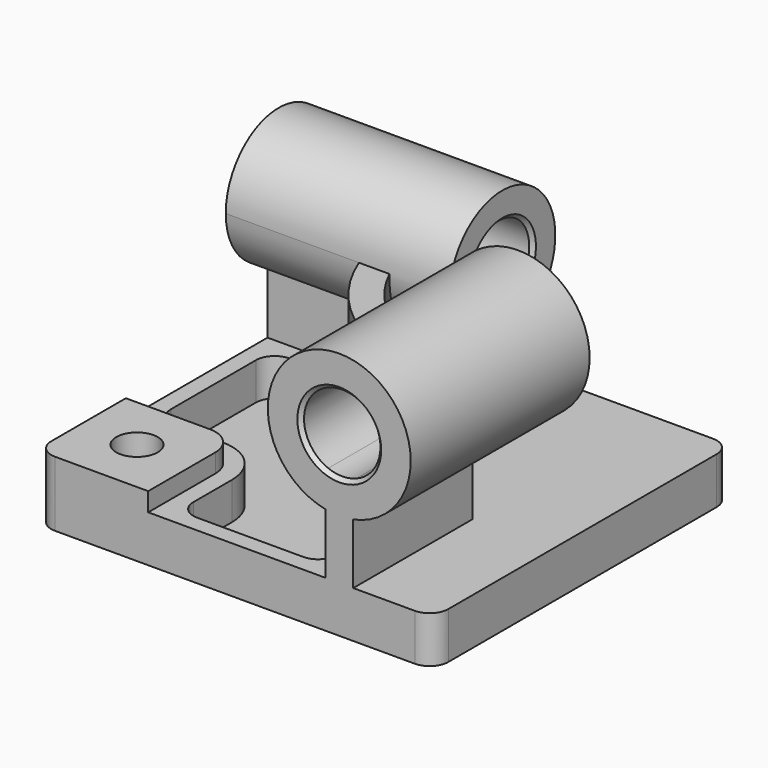
from build123d import *

# Parameters (mm, degrees)
F0_W            = 213
F0_H            = 25
F1_DEPTH        = 100
F3_DEPTH        = 20
F4_DEPTH        = 70
F5_R            = 38.333333335
F5_R_2          = 20.5
F6_DEPTH        = 120
F7_R            = 35.5
F7_R_2          = 20.5
F8_DEPTH        = 120
F9_DEPTH        = 213.001
F10_DEPTH       = 200.001
F11_DEPTH       = 10
F13_D           = 14.75
F13_CBORE_D     = 22.25
F13_CBORE_DEPTH = 14
F14_R           = 10


# Not quite as in the source:
# - a fillet or chamfer that OpenCascade refuses, or shapes differently, is made with other operations: its cross-section is extruded or revolved along the edge and cut away or added


with BuildPart() as f1:
    # F0 (on Front) → F1 (new body, symmetric)
    with BuildSketch(Plane.XZ):
        with Locations((0, 12.5)):
            Rectangle(F0_W, F0_H)
    extrude(amount=F1_DEPTH, both=True)

    # F2 (on face) → F3 (cut)
    with BuildSketch(Plane.XY.offset(25)):
        with BuildLine():
            ThreePointArc((-97.5, -21), (-94.5710678119, -28.0710678119), (-87.5, -31))
            Line((-87.5, -31), (-61.5, -31))
            ThreePointArc((-61.5, -31), (-44.5294372515, -38.0294372515), (-37.5, -55))
            Line((-37.5, -55), (-37.5, -81))
            ThreePointArc((-37.5, -81), (-34.5710678119, -88.0710678119), (-27.5, -91))
            Line((-27.5, -91), (29.5, -91))
            ThreePointArc((29.5, -91), (36.5710678119, -88.0710678119), (39.5, -81))
            Line((39.5, -81), (39.5, -51.2013330404))
            ThreePointArc((39.5, -51.2013330404), (37.338740663, -44.9921346366), (31.7891710363, -41.4668738378))
            ThreePointArc((31.7891710363, -41.4668738378), (-19.4358675785, -12.9358675785), (-47.9668738378, 38.2891710363))
            ThreePointArc((-47.9668738378, 38.2891710363), (-51.4921346366, 43.838740663), (-57.7013330404, 46))
            Line((-57.7013330404, 46), (-87.5, 46))
            ThreePointArc((-87.5, 46), (-94.5710678119, 43.0710678119), (-97.5, 36))
            Line((-97.5, 36), (-97.5, -21))
        make_face()
    extrude(amount=-F3_DEPTH, mode=Mode.SUBTRACT)

    # F2 (on face) → F4 (join)
    with BuildSketch(Plane.XY.offset(25)):
        with BuildLine():
            Line((-26.5, 70), (-106.5, 70))
            Line((-106.5, 70), (-106.5, 55))
            Line((-106.5, 55), (-41.5, 55))
            ThreePointArc((-41.5, 55), (-13.0719065478, -6.5719065478), (48.5, -35))
            Line((48.5, -35), (48.5, -100))
            Line((48.5, -100), (63.5, -100))
            Line((63.5, -100), (63.5, -20))
            ThreePointArc((63.5, -20), (-2.46530483, 4.03469517), (-26.5, 70))
        make_face()
    extrude(amount=F4_DEPTH)

    # F5 (on face) → F6 (join)
    with BuildSketch(Plane.XZ.offset(100)):
        with Locations((56, 95)):
            Circle(F5_R)
        with Locations((56, 95)):
            Circle(F5_R_2, mode=Mode.SUBTRACT)
    extrude(amount=-F6_DEPTH)

    # F7 (on face) → F8 (join)
    with BuildSketch(Plane(origin=(-106.5, 0, 0), x_dir=(0, -1, 0), z_dir=(-1, 0, 0))):
        with Locations((-62.5, 95)):
            Circle(F7_R)
        with Locations((-62.5, 95)):
            Circle(F7_R_2, mode=Mode.SUBTRACT)
    extrude(amount=-F8_DEPTH)

    # F7 (on face) → F9 (cut, through all)
    with BuildSketch(Plane(origin=(-106.5, 0, 0), x_dir=(0, -1, 0), z_dir=(-1, 0, 0))):
        with BuildLine():
            ThreePointArc((-42, 95), (-74.0433963806, 111.9410743461), (-70, 75.9212159717))
            Line((-70, 75.9212159717), (-70, 95))
            Line((-70, 95), (-55, 95))
            Line((-55, 95), (-55, 75.9212159717))
            ThreePointArc((-55, 75.9212159717), (-45.5589256539, 83.4566036194), (-42, 95))
        make_face()
        with BuildLine():
            Line((-70, 95), (-70, 75.9212159717))
            ThreePointArc((-70, 75.9212159717), (-62.5, 74.5), (-55, 75.9212159717))
            Line((-55, 75.9212159717), (-55, 95))
            Line((-55, 95), (-70, 95))
        make_face()
    extrude(amount=-F9_DEPTH, mode=Mode.SUBTRACT)

    # F5 (on face) → F10 (cut, through all)
    with BuildSketch(Plane.XZ.offset(100)):
        with BuildLine():
            ThreePointArc((76.5, 95), (44.4566036194, 111.9410743461), (48.5, 75.9212159717))
            Line((48.5, 75.9212159717), (48.5, 95))
            Line((48.5, 95), (63.5, 95))
            Line((63.5, 95), (63.5, 75.9212159717))
            ThreePointArc((63.5, 75.9212159717), (72.9410743461, 83.4566036194), (76.5, 95))
        make_face()
        with BuildLine():
            Line((48.5, 95), (48.5, 75.9212159717))
            ThreePointArc((48.5, 75.9212159717), (56, 74.5), (63.5, 75.9212159717))
            Line((63.5, 75.9212159717), (63.5, 95))
            Line((63.5, 95), (48.5, 95))
        make_face()
    extrude(amount=-F10_DEPTH, mode=Mode.SUBTRACT)

    # F2 (on face) → F11 (join)
    with BuildSketch(Plane.XY.offset(25)):
        with BuildLine():
            Line((-61.5, -40), (-106.5, -40))
            Line((-106.5, -40), (-106.5, -100))
            Line((-106.5, -100), (-46.5, -100))
            Line((-46.5, -100), (-46.5, -55))
            ThreePointArc((-46.5, -55), (-50.8933982822, -44.3933982822), (-61.5, -40))
        make_face()
    extrude(amount=F11_DEPTH)

    # F13 (through all)
    with Locations(Plane.XY.offset(35)):
        with Locations((-76.5, -70)):
            CounterBoreHole(F13_D / 2, F13_CBORE_D / 2, F13_CBORE_DEPTH)

    # F14
    f14_edges = [f1.edges().sort_by_distance(p)[0] for p in [
        (106.5, -100, 12.5),
        (106.5, 100, 12.5),
        (-106.5, 100, 12.5),
        (-106.5, -100, 17.5),
    ]]
    fillet(f14_edges, radius=F14_R)

    # F15: chamfer of 2 on 4 edges, made by hand

    # F15_s1 → F15_t2 (revolve, cut)
    with BuildSketch(Plane.XY.offset(95)):
        Polygon((78.5, -100), (76.5, -98), (76.5, -100), align=None)
    revolve(axis=Axis((56, -100, 95), (0, 1, 0)), mode=Mode.SUBTRACT)

    # F15_s3 → F15_t4 (revolve, cut)
    with BuildSketch(Plane.XY.offset(95)):
        Polygon((-106.5, 40), (-104.5, 42), (-106.5, 42), align=None)
    revolve(axis=Axis((-106.5, 62.5, 95), (1, 0, 0)), mode=Mode.SUBTRACT)

    # F15_s5 → F15_t6 (revolve, cut)
    with BuildSketch(Plane.XY.offset(95)):
        Polygon((11.5, 42), (13.5, 40), (13.5, 42), align=None)
    revolve(axis=Axis((13.5, 62.5, 95), (-1, 0, 0)), mode=Mode.SUBTRACT)

    # F15_s7 → F15_t8 (revolve, cut)
    with BuildSketch(Plane.XY.offset(95)):
        Polygon((76.5, 18), (78.5, 20), (76.5, 20), align=None)
    revolve(axis=Axis((56, 20, 95), (0, -1, 0)), mode=Mode.SUBTRACT)


solid = f1.part
